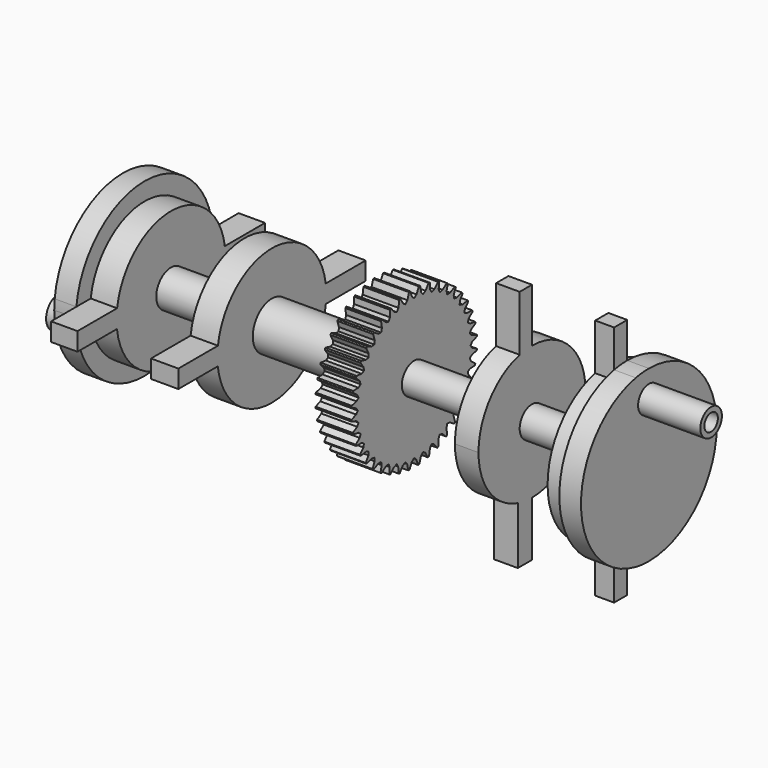
from build123d import *

# Parameters (mm, degrees)
F1_DEPTH  = 5.08
F3_DEPTH  = 5.842
F5_R      = 4.1520133517
F6_DEPTH  = 26.924
F7_R      = 4.1520133517
F8_DEPTH  = 6.35
F9_R      = 4.1476855986
F10_DEPTH = 25.4
F11_W     = 84.2210557312
F11_H     = 11.4299990237
F11_W_2   = 84.8226295784
F11_H_2   = 20.7544751465
F12_DEPTH = 13.208
F13_R     = 21.1650894072
F13_R_2   = 4.1476855986
F14_DEPTH = 9.652
F16_DEPTH = 25.4
F17_COUNT = 40
F18_R     = 6.4114387171
F19_DEPTH = 28.702
F20_R     = 6.4114387171
F21_DEPTH = 6.604
F22_DEPTH = 7.366
F23_R     = 4.9462001283
F24_DEPTH = 19.812
F25_R     = 4.9462001283
F26_DEPTH = 7.112
F28_DEPTH = 5.842
F29_R     = 3.6385680332
F29_R_2   = 2.2751870905
F30_DEPTH = 7.62
F31_R     = 4.2750225612
F31_R_2   = 2.7731432897
F32_DEPTH = 4.572
F33_DEPTH = 12.7
F34_DEPTH = 9.144


# Not quite as in the source:
# - a feature names something its author has since deleted; it is built from what else it names


with BuildPart() as f1:
    # F0 (on Right) → F1 (new body)
    with BuildSketch(Plane.YZ):
        with BuildLine():
            ThreePointArc((0, -20.4708488309), (14.4750760249, -14.4750760249), (20.4708488309, 0))
            ThreePointArc((20.4708488309, 0), (14.4750760249, 14.4750760249), (0, 20.4708488309))
            ThreePointArc((0, 20.4708488309), (-2.2257968393, 20.3494835386), (-4.425201565, 19.9868267358))
            ThreePointArc((-4.425201565, 19.9868267358), (-20.4708488309, 0), (-4.425201565, -19.9868267358))
            ThreePointArc((-4.425201565, -19.9868267358), (-2.2257968393, -20.3494835386), (0, -20.4708488309))
        make_face()
        with BuildLine():
            ThreePointArc((-4.425201565, 19.9868267358), (-2.2257968393, 20.3494835386), (0, 20.4708488309))
            Line((0, 20.4708488309), (0, 32.8725613654))
            Line((0, 32.8725613654), (-4.425201565, 32.8138524732))
            Line((-4.425201565, 32.8138524732), (-4.425201565, 19.9868267358))
        make_face()
        with BuildLine():
            Line((0, -32.8725613654), (0, -20.4708488309))
            ThreePointArc((0, -20.4708488309), (-2.2257968393, -20.3494835386), (-4.425201565, -19.9868267358))
            Line((-4.425201565, -19.9868267358), (-4.425201565, -32.8138524732))
            Line((-4.425201565, -32.8138524732), (0, -32.8725613654))
        make_face()
    extrude(amount=F1_DEPTH)

    # F2 (on face) → F3 (join)
    with BuildSketch(Plane.YZ.offset(5.08)):
        with BuildLine():
            ThreePointArc((0, -22.8645966633), (16.1677113497, -16.1677113497), (22.8645966633, 0))
            ThreePointArc((22.8645966633, 0), (16.1677113497, 16.1677113497), (0, 22.8645966633))
            Line((0, 22.8645966633), (0, 20.4708488309))
            ThreePointArc((0, 20.4708488309), (20.4708488309, 0), (0, -20.4708488309))
            Line((0, -20.4708488309), (0, -22.8645966633))
        make_face()
        with BuildLine():
            Line((0, 20.4708488309), (0, 22.8645966633))
            ThreePointArc((0, 22.8645966633), (-2.2231342183, 22.7562618816), (-4.425201565, 22.4322841388))
            Line((-4.425201565, 22.4322841388), (-4.425201565, 19.9868267358))
            ThreePointArc((-4.425201565, 19.9868267358), (-20.4708488309, 0), (-4.425201565, -19.9868267358))
            Line((-4.425201565, -19.9868267358), (-4.425201565, -22.4322841388))
            ThreePointArc((-4.425201565, -22.4322841388), (-2.2231342183, -22.7562618816), (0, -22.8645966633))
            Line((0, -22.8645966633), (0, -20.4708488309))
            ThreePointArc((0, -20.4708488309), (20.4708488309, 0), (0, 20.4708488309))
        make_face()
        with BuildLine():
            Line((-4.425201565, 19.9868267358), (-4.425201565, 22.4322841388))
            ThreePointArc((-4.425201565, 22.4322841388), (-22.8645966633, 0), (-4.425201565, -22.4322841388))
            Line((-4.425201565, -22.4322841388), (-4.425201565, -19.9868267358))
            ThreePointArc((-4.425201565, -19.9868267358), (-20.4708488309, 0), (-4.425201565, 19.9868267358))
        make_face()
    extrude(amount=F3_DEPTH)

    # F5 (on face) → F6 (join)
    with BuildSketch(Plane(origin=(0, 0, 0), x_dir=(0, -1, 0), z_dir=(-1, 0, 0))):
        Circle(F5_R)
    extrude(amount=F6_DEPTH)

    # F7 (on face) → F8 (join)
    with BuildSketch(Plane(origin=(-26.924, 0, 0), x_dir=(0, -1, 0), z_dir=(-1, 0, 0))):
        with BuildLine():
            ThreePointArc((4.7857561149, -17.3808329088), (14.3400285329, -10.9252183442), (18.0276680187, 0))
            ThreePointArc((18.0276680187, 0), (14.1380676404, 11.1853411923), (4.1476855986, 17.5440450971))
            ThreePointArc((4.1476855986, 17.5440450971), (2.0878928945, 17.9063541084), (0, 18.0276680187))
            ThreePointArc((0, 18.0276680187), (-18.0276680187, 0), (0, -18.0276680187))
            ThreePointArc((0, -18.0276680187), (2.4146354409, -17.8652273952), (4.7857561149, -17.3808329088))
        make_face()
        Circle(F7_R, mode=Mode.SUBTRACT)
        with BuildLine():
            ThreePointArc((0, 18.0276680187), (2.0878928945, 17.9063541084), (4.1476855986, 17.5440450971))
            Line((4.1476855986, 17.5440450971), (4.1476855986, 42.3946790397))
            Line((4.1476855986, 42.3946790397), (0, 39.4170172513))
            Line((0, 39.4170172513), (0, 18.0276680187))
        make_face()
        with BuildLine():
            Line((4.7857561149, -37.1514819562), (4.7857561149, -17.3808329088))
            ThreePointArc((4.7857561149, -17.3808329088), (2.4146354409, -17.8652273952), (0, -18.0276680187))
            Line((0, -18.0276680187), (0, -39.4910760224))
            Line((0, -39.4910760224), (4.7857561149, -37.1514819562))
        make_face()
    extrude(amount=-F8_DEPTH)

    # F9 (on face) → F10 (join)
    with BuildSketch(Plane(origin=(-26.924, 0, 0), x_dir=(0, -1, 0), z_dir=(-1, 0, 0))):
        Circle(F9_R)
    extrude(amount=F10_DEPTH)

    # F11 (on Front) → F12 (cut)
    with BuildSketch(Plane.XZ):
        with Locations((-29.9285547808, 38.2002647966)):
            Rectangle(F11_W, F11_H)
        with Locations((-28.1238160096, -43.1632902473)):
            Rectangle(F11_W_2, F11_H_2)
    extrude(amount=F12_DEPTH, mode=Mode.SUBTRACT)

    # F13 (on face) → F14 (join)
    with BuildSketch(Plane(origin=(-52.324, 0, 0), x_dir=(0, -1, 0), z_dir=(-1, 0, 0))):
        Circle(F13_R)
        Circle(F13_R_2, mode=Mode.SUBTRACT)
        Circle(F13_R_2)
    extrude(amount=F14_DEPTH)

    # F15 (on face) → F16 (cut)
    with BuildSketch(Plane(origin=(-61.976, 0, 0), x_dir=(0, -1, 0), z_dir=(-1, 0, 0))):
        with BuildLine():
            ThreePointArc((1.310742254, 21.1244636466), (-0.1339755114, 21.1646653689), (-1.5780685539, 21.1061770402))
            Line((-1.5780685539, 21.1061770402), (-0.7766649942, 19.5370744914))
            Line((-0.7766649942, 19.5370744914), (0, 18.9521759748))
            Line((0, 18.9521759748), (0.6955460995, 19.5370744914))
            Line((0.6955460995, 19.5370744914), (1.310742254, 21.1244636466))
        make_face()
    f16 = extrude(amount=-F16_DEPTH, mode=Mode.SUBTRACT)

    # F17: F16 ×40 about axis
    f17_axis = Axis((-52.324, 0, 0), (1, 0, 0))
    for i in range(1, F17_COUNT):
        add(f16.rotate(f17_axis, i * 360 / F17_COUNT), mode=Mode.SUBTRACT)

    # F18 (on face) → F19 (join)
    with BuildSketch(Plane(origin=(-61.976, 0, 0), x_dir=(0, -1, 0), z_dir=(-1, 0, 0))):
        Circle(F18_R)
    extrude(amount=F19_DEPTH)

    # F20 (on face) → F21 (join)
    with BuildSketch(Plane(origin=(-90.678, 0, 0), x_dir=(0, -1, 0), z_dir=(-1, 0, 0))):
        with BuildLine():
            ThreePointArc((18.1928136018, -2.2680452093), (18.2984023965, -1.1362066518), (18.3336438228, 0))
            ThreePointArc((18.3336438228, 0), (18.2874517996, 1.3006162002), (18.1491084935, 2.5946785375))
            ThreePointArc((18.1491084935, 2.5946785375), (0, 18.3336438228), (-18.1491084935, 2.5946785375))
            ThreePointArc((-18.1491084935, 2.5946785375), (-18.3329033695, 0.1647721666), (-18.1928136018, -2.2680452093))
            ThreePointArc((-18.1928136018, -2.2680452093), (0, -18.3336438228), (18.1928136018, -2.2680452093))
        make_face()
        Circle(F20_R, mode=Mode.SUBTRACT)
        Circle(F20_R)
    extrude(amount=F21_DEPTH)

    # F20 (on face) → F22 (join)
    with BuildSketch(Plane(origin=(-90.678, 0, 0), x_dir=(0, -1, 0), z_dir=(-1, 0, 0))):
        with BuildLine():
            ThreePointArc((18.1928136018, -2.2680452093), (18.2984023965, -1.1362066518), (18.3336438228, 0))
            ThreePointArc((18.3336438228, 0), (18.2874517996, 1.3006162002), (18.1491084935, 2.5946785375))
            ThreePointArc((18.1491084935, 2.5946785375), (0, 18.3336438228), (-18.1491084935, 2.5946785375))
            ThreePointArc((-18.1491084935, 2.5946785375), (-18.3329033695, 0.1647721666), (-18.1928136018, -2.2680452093))
            ThreePointArc((-18.1928136018, -2.2680452093), (0, -18.3336438228), (18.1928136018, -2.2680452093))
        make_face()
        with BuildLine():
            ThreePointArc((18.1491084935, 2.5946785375), (18.2874517996, 1.3006162002), (18.3336438228, 0))
            ThreePointArc((18.3336438228, 0), (18.2984023965, -1.1362066518), (18.1928136018, -2.2680452093))
            Line((18.1928136018, -2.2680452093), (31.4867012203, -2.2680452093))
            Line((31.4867012203, -2.2680452093), (31.4867012203, 0))
            Line((31.4867012203, 0), (31.4867012203, 2.5946785375))
            Line((31.4867012203, 2.5946785375), (18.1491084935, 2.5946785375))
        make_face()
        with BuildLine():
            ThreePointArc((-18.1928136018, -2.2680452093), (-18.3329033695, 0.1647721666), (-18.1491084935, 2.5946785375))
            Line((-18.1491084935, 2.5946785375), (-31.6057130694, 2.5946785375))
            Line((-31.6057130694, 2.5946785375), (-31.6057130694, 0))
            Line((-31.6057130694, 0), (-31.6057130694, -2.2680452093))
            Line((-31.6057130694, -2.2680452093), (-18.1928136018, -2.2680452093))
        make_face()
    extrude(amount=F22_DEPTH)

    # F23 (on face) → F24 (join)
    with BuildSketch(Plane(origin=(-98.044, 0, 0), x_dir=(0, -1, 0), z_dir=(-1, 0, 0))):
        Circle(F23_R)
    extrude(amount=F24_DEPTH)

    # F25 (on face) → F26 (join)
    with BuildSketch(Plane(origin=(-117.856, 0, 0), x_dir=(0, -1, 0), z_dir=(-1, 0, 0))):
        with BuildLine():
            ThreePointArc((18.1856173017, -2.2592737805), (18.2904354514, -1.1317975338), (18.3254193583, 0))
            ThreePointArc((18.3254193583, 0), (18.2775592124, 1.3235648444), (18.1342287653, 2.6402162311))
            ThreePointArc((18.1342287653, 2.6402162311), (-0.0038469595, 18.3254189546), (-18.1353356606, 2.6326023508))
            ThreePointArc((-18.1353356606, 2.6326023508), (-18.3243779894, 0.1953610999), (-18.1873408867, -2.2453565711))
            ThreePointArc((-18.1873408867, -2.2453565711), (-0.0070117663, -18.3254180169), (18.1856173017, -2.2592737805))
        make_face()
        Circle(F25_R, mode=Mode.SUBTRACT)
        Circle(F25_R)
        with BuildLine():
            ThreePointArc((-18.1873408867, -2.2453565711), (-18.3243779894, 0.1953610999), (-18.1353356606, 2.6326023508))
            Line((-18.1353356606, 2.6326023508), (-31.6914805857, 2.6326023508))
            Line((-31.6914805857, 2.6326023508), (-31.6914805857, -2.2453565711))
            Line((-31.6914805857, -2.2453565711), (-18.1873408867, -2.2453565711))
        make_face()
        with BuildLine():
            ThreePointArc((18.1342287653, 2.6402162311), (18.2775592124, 1.3235648444), (18.3254193583, 0))
            ThreePointArc((18.3254193583, 0), (18.2904354514, -1.1317975338), (18.1856173017, -2.2592737805))
            Line((18.1856173017, -2.2592737805), (31.477529748, -2.2592737805))
            Line((31.477529748, -2.2592737805), (31.477529748, 2.6402162311))
            Line((31.477529748, 2.6402162311), (18.1342287653, 2.6402162311))
        make_face()
    extrude(amount=F26_DEPTH)

    # F27 (on face) → F28 (join)
    with BuildSketch(Plane(origin=(-124.968, 0, 0), x_dir=(0, -1, 0), z_dir=(-1, 0, 0))):
        with BuildLine():
            ThreePointArc((-23.0065128899, -2.2453565711), (-0.0069918736, -23.1158216942), (23.0051503683, -2.2592737805))
            Line((23.0051503683, -2.2592737805), (18.1856173017, -2.2592737805))
            ThreePointArc((18.1856173017, -2.2592737805), (-0.0070117663, -18.3254180169), (-18.1873408867, -2.2453565711))
            Line((-18.1873408867, -2.2453565711), (-23.0065128899, -2.2453565711))
        make_face()
        with BuildLine():
            ThreePointArc((23.0051503683, -2.2592737805), (23.0881380775, -1.1309914226), (23.1158227516, 0))
            ThreePointArc((23.1158227516, 0), (23.0779733756, 1.3222731786), (22.9645491952, 2.6402162311))
            Line((22.9645491952, 2.6402162311), (18.1342287653, 2.6402162311))
            ThreePointArc((18.1342287653, 2.6402162311), (-0.0038469595, 18.3254189546), (-18.1353356606, 2.6326023508))
            Line((-18.1353356606, 2.6326023508), (-22.9654232782, 2.6326023508))
            ThreePointArc((-22.9654232782, 2.6326023508), (-23.1150026946, 0.1947098162), (-23.0065128899, -2.2453565711))
            Line((-23.0065128899, -2.2453565711), (-18.1873408867, -2.2453565711))
            ThreePointArc((-18.1873408867, -2.2453565711), (-0.0070117663, -18.3254180169), (18.1856173017, -2.2592737805))
            Line((18.1856173017, -2.2592737805), (23.0051503683, -2.2592737805))
        make_face()
        with BuildLine():
            Line((18.1342287653, 2.6402162311), (22.9645491952, 2.6402162311))
            ThreePointArc((22.9645491952, 2.6402162311), (-0.0038319445, 23.115822434), (-22.9654232782, 2.6326023508))
            Line((-22.9654232782, 2.6326023508), (-18.1353356606, 2.6326023508))
            ThreePointArc((-18.1353356606, 2.6326023508), (-0.0038469595, 18.3254189546), (18.1342287653, 2.6402162311))
        make_face()
    extrude(amount=F28_DEPTH)

    # F29 (on face) → F30 (join)
    with BuildSketch(Plane.YZ.offset(10.922)):
        with Locations((0, 15.5682079494)):
            Circle(F29_R)
        with Locations((0, 15.5682079494)):
            Circle(F29_R_2, mode=Mode.SUBTRACT)
    extrude(amount=F30_DEPTH)

    # F31 (on face) → F32 (join)
    with BuildSketch(Plane(origin=(-130.81, 0, 0), x_dir=(0, -1, 0), z_dir=(-1, 0, 0))):
        with Locations((0, -15.340263024)):
            Circle(F31_R)
        with Locations((0, -15.340263024)):
            Circle(F31_R_2, mode=Mode.SUBTRACT)
    extrude(amount=F32_DEPTH)

    # F33 (add): a face of the model
    f33_faces = [f1.faces().sort_by_distance(p)[0] for p in [
        (-135.382, 4.1541066635, -15.340263024),
    ]]
    extrude(f33_faces, amount=F33_DEPTH)

    # F34 (add): a face of the model
    f34_faces = [f1.faces().sort_by_distance(p)[0] for p in [
        (18.542, -3.535653788, 15.5682079494),
    ]]
    extrude(f34_faces, amount=F34_DEPTH)


solid = f1.part
